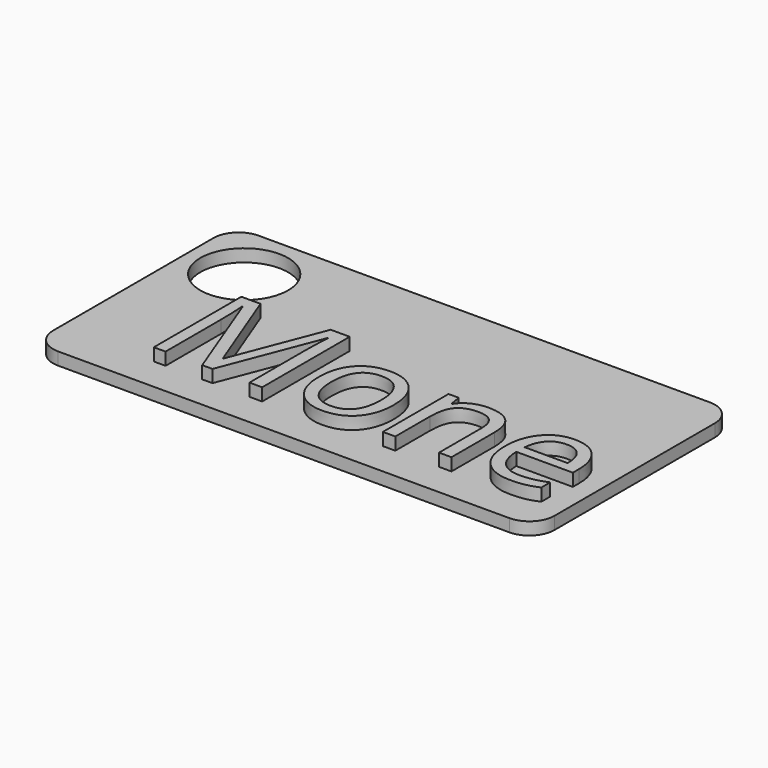
from build123d import *

# Parameters (mm, degrees)
F0_W         = 40
F0_H         = 20
F1_DEPTH     = 1
F2_TEXT_SIZE = 12.2282612008
F3_DEPTH     = 1
F5_R         = 2
F6_D         = 7
F6_DEPTH     = 50
F6_TIP       = 2.1030121666


# Not quite as in the source:
# - Text() gives the source's letters only with a copy of the font that has no kerning and outlines rounded to 1/6400 em; it was checked with that copy


with BuildPart() as f1:
    # F0 (on Top) → F1 (new body)
    with BuildSketch(Plane.XY):
        Rectangle(F0_W, F0_H)
    extrude(amount=F1_DEPTH)

    # F2 (on face) → F3 (join)
    with BuildSketch(Plane.XY.offset(1)):
        with Locations((-13.6956572533, -7.3369567981)):
            Text('Mone', F2_TEXT_SIZE, font='Open Sans', text_align=(TextAlign.LEFT, TextAlign.BOTTOM))
    extrude(amount=F3_DEPTH)

    # F5
    f5_edges = [f1.edges().sort_by_distance(p)[0] for p in [
        (-20, 10, 0.5),
        (-20, -10, 0.5),
        (20, -10, 0.5),
        (20, 10, 0.5),
    ]]
    fillet(f5_edges, radius=F5_R)

    # F6
    with Locations(Plane.XY.offset(1)):
        with Locations((-15.4565228149, 5.3804349154)):
            Hole(F6_D / 2, depth=F6_DEPTH)
            with Locations((0, 0, -(F6_DEPTH + F6_TIP / 2))):  # 118° drill point
                Cone(0, F6_D / 2, F6_TIP, mode=Mode.SUBTRACT)


solid = f1.part
